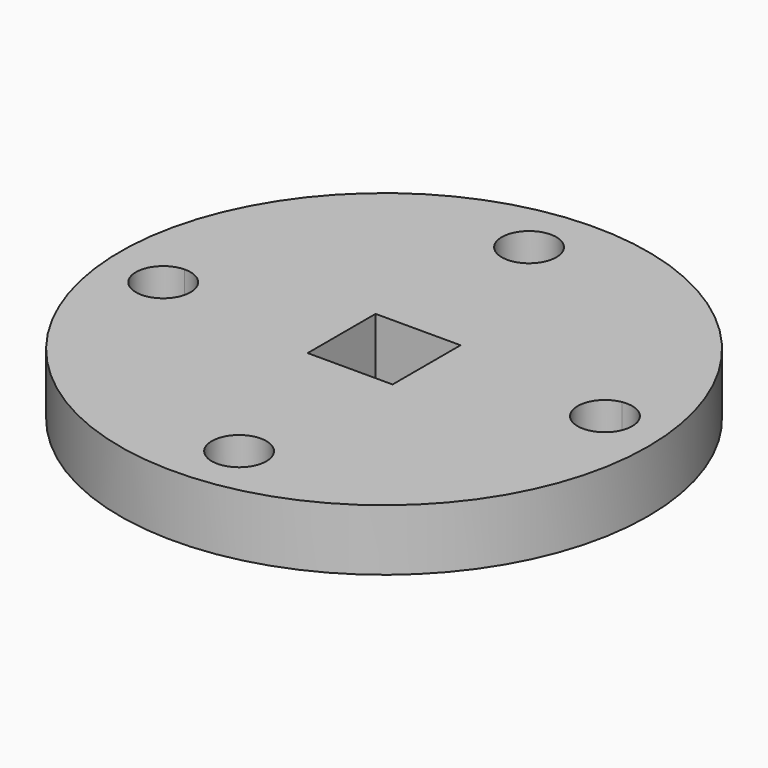
from build123d import *

# Parameters (mm, degrees)
F0_R     = 1104.9
F0_W     = 355.6
F0_H     = 355.6
F1_DEPTH = 256.54
F3_DEPTH = 711.2


# Not quite as in the source:
# - a feature of the source that left no trace in its solid (it failed there, or was rolled back) is left out


with BuildPart() as f1:
    # F0 (on Top) → F1 (new body)
    with BuildSketch(Plane.XY):
        Circle(F0_R)
        Rectangle(F0_W, F0_H, mode=Mode.SUBTRACT)
    extrude(amount=F1_DEPTH)

    # F2 (on face) → F3 (cut)
    with BuildSketch(Plane.XY.offset(256.54)):
        with BuildLine():
            ThreePointArc((33.3315313944, 862.9565278824), (-80.9248760483, 859.8000491024), (-193.7636980758, 841.5821940298))
            ThreePointArc((-193.7636980758, 841.5821940298), (-71.7866967368, 745.8659291959), (33.3751239517, 859.8000491024))
            ThreePointArc((33.3751239517, 859.8000491024), (33.3642252927, 861.378438994), (33.3315313944, 862.9565278824))
        make_face()
        with BuildLine():
            ThreePointArc((33.3315313944, 862.9565278824), (-91.6355214077, 973.5971144248), (-193.7636980758, 841.5821940298))
            ThreePointArc((-193.7636980758, 841.5821940298), (-80.9248760483, 859.8000491024), (33.3315313944, 862.9565278824))
        make_face()
        with BuildLine():
            ThreePointArc((-841.5821940298, -193.7636980758), (-858.07789354, -97.5053261004), (-863.6, 0))
            Line((-863.6, 0), (-940.5196528958, 0))
            ThreePointArc((-940.5196528958, 0), (-961.597445048, -132.9035272304), (-841.5821940298, -193.7636980758))
        make_face()
        with BuildLine():
            ThreePointArc((-745.5000491024, -80.9248760483), (-754.2284129647, -37.1171182513), (-779.0804453091, 0))
            Line((-779.0804453091, 0), (-863.6, 0))
            ThreePointArc((-863.6, 0), (-858.07789354, -97.5053261004), (-841.5821940298, -193.7636980758))
            ThreePointArc((-841.5821940298, -193.7636980758), (-772.7747917492, -155.0267962839), (-745.5000491024, -80.9248760483))
        make_face()
        with BuildLine():
            ThreePointArc((974.1000491024, 80.9248760483), (933.901969338, 167.9501334016), (841.5821940298, 193.7636980758))
            ThreePointArc((841.5821940298, 193.7636980758), (858.07789354, 97.5053261004), (863.6, 0))
            ThreePointArc((863.6, 0), (863.4391169849, -16.6688709985), (862.9565278824, -33.3315313944))
            ThreePointArc((862.9565278824, -33.3315313944), (941.7307378721, 1.2263676701), (974.1000491024, 80.9248760483))
        make_face()
        with BuildLine():
            ThreePointArc((863.6, 0), (858.07789354, 97.5053261004), (841.5821940298, 193.7636980758))
            ThreePointArc((841.5821940298, 193.7636980758), (746.0029837801, 70.214230689), (862.9565278824, -33.3315313944))
            ThreePointArc((862.9565278824, -33.3315313944), (863.4391169849, -16.6688709985), (863.6, 0))
        make_face()
        with BuildLine():
            ThreePointArc((193.7636980758, -841.5821940298), (80.9248760483, -859.8000491024), (-33.3315313944, -862.9565278824))
            ThreePointArc((-33.3315313944, -862.9565278824), (82.5032659399, -974.0891504435), (195.2248760483, -859.8000491024))
            ThreePointArc((195.2248760483, -859.8000491024), (194.8589959549, -850.661869791), (193.7636980758, -841.5821940298))
        make_face()
        with BuildLine():
            ThreePointArc((193.7636980758, -841.5821940298), (70.214230689, -746.0029837801), (-33.3315313944, -862.9565278824))
            ThreePointArc((-33.3315313944, -862.9565278824), (80.9248760483, -859.8000491024), (193.7636980758, -841.5821940298))
        make_face()
        with BuildLine():
            Line((-940.5196528958, 0), (-863.6, 0))
            ThreePointArc((-863.6, 0), (-863.4391169849, 16.6688709985), (-862.9565278824, 33.3315313944))
            ThreePointArc((-862.9565278824, 33.3315313944), (-904.9281673131, 24.0891370488), (-940.5196528958, 0))
        make_face()
        with BuildLine():
            Line((-863.6, 0), (-779.0804453091, 0))
            ThreePointArc((-779.0804453091, 0), (-817.5891815831, 25.295332308), (-862.9565278824, 33.3315313944))
            ThreePointArc((-862.9565278824, 33.3315313944), (-863.4391169849, 16.6688709985), (-863.6, 0))
        make_face()
    extrude(amount=-F3_DEPTH, mode=Mode.SUBTRACT)


solid = f1.part
